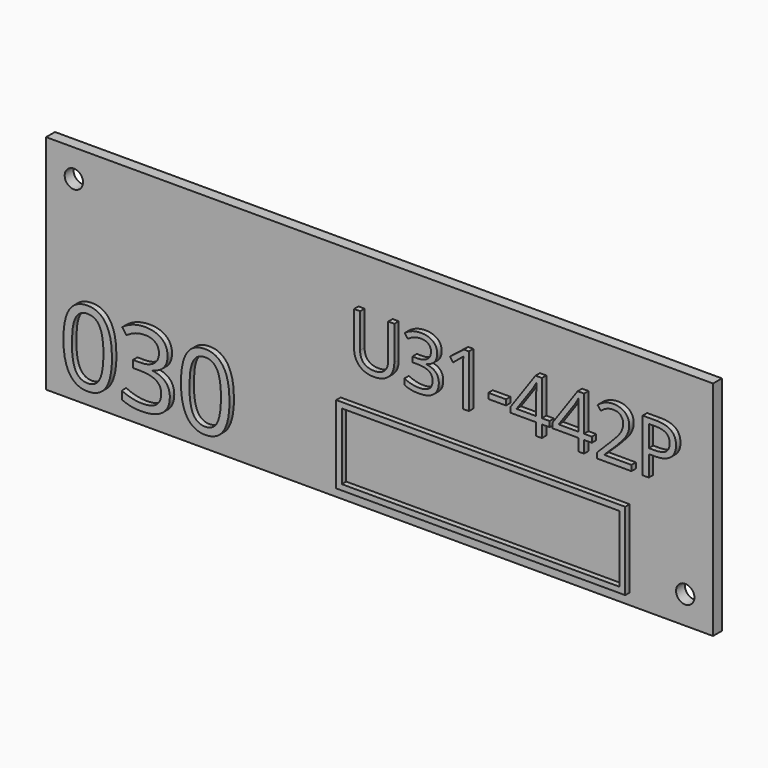
from build123d import *

# Parameters (mm, degrees)
F0_W         = 120
F0_H         = 40
F1_DEPTH     = 2
F3_D         = 3.3
F4_TEXT_SIZE = 13.2628743135
F5_DEPTH     = 1
F6_TEXT_SIZE = 18.4937691891
F7_DEPTH     = 1
F8_W         = 52
F8_H         = 14
F8_W_2       = 49.99999962
F8_H_2       = 11.99999962
F9_DEPTH     = 1


# Not quite as in the source:
# - Text() gives the source's letters only with a copy of the font that has no kerning and outlines rounded to 1/6400 em; it was checked with that copy


with BuildPart() as f1:
    # F0 (on Front) → F1 (new body)
    with BuildSketch(Plane.XZ):
        Rectangle(F0_W, F0_H)
    extrude(amount=F1_DEPTH)

    # F3 (through all)
    with Locations(Plane.XZ.offset(2)):
        with Locations((-55, 15), (55, -15)):
            Hole(F3_D / 2)

    # F4 (on face) → F5 (join)
    with BuildSketch(Plane.XZ.offset(2)):
        with Locations((-5, 2)):
            Text('U31-442P', F4_TEXT_SIZE, font='Open Sans', text_align=(TextAlign.LEFT, TextAlign.BOTTOM))
    extrude(amount=F5_DEPTH)

    # F6 (on face) → F7 (join)
    with BuildSketch(Plane.XZ.offset(2)):
        with Locations((-57, -17)):
            Text('030', F6_TEXT_SIZE, font='Open Sans', text_align=(TextAlign.LEFT, TextAlign.BOTTOM))
    extrude(amount=F7_DEPTH)

    # F8 (on face) → F9 (join)
    with BuildSketch(Plane.XZ.offset(2)):
        with Locations((19, -11)):
            Rectangle(F8_W, F8_H)
        with Locations((19, -11)):
            Rectangle(F8_W_2, F8_H_2, mode=Mode.SUBTRACT)
    extrude(amount=F9_DEPTH)


solid = f1.part
